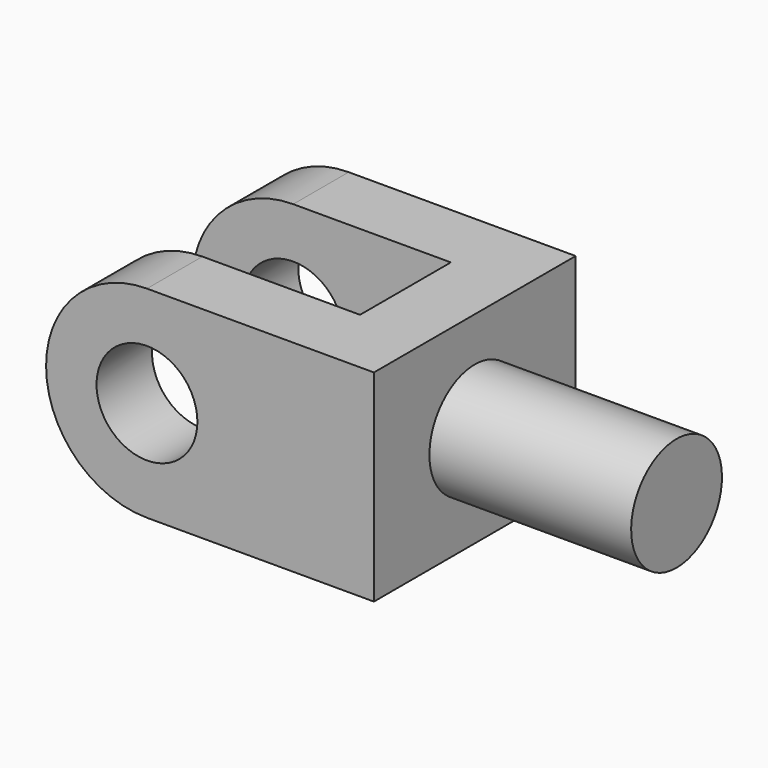
from build123d import *

# Parameters (mm, degrees)
F1_DEPTH = 812.8
F2_R     = 406.39999
F3_R     = 203.2
F4_DEPTH = 1016.001
F6_DEPTH = 812.8


# Not quite as in the source:
# - a fillet or chamfer is up to 0.001 mm smaller than in the source, because OpenCascade refuses the exact size


with BuildPart() as f1:
    # F0 (on Top) → F1 (new body)
    with BuildSketch(Plane.XY):
        Polygon((-69.4132745266, 217.2510341048), (-69.4132745266, -62.1489658952), (1251.3867254734, -62.1489658952), (1251.3867254734, 953.8510341048), (-69.4132745266, 953.8510341048), (-69.4132745266, 674.4510341048), (971.9867254734, 674.4510341048), (971.9867254734, 217.2510341048), align=None)
    extrude(amount=F1_DEPTH)

    # F2 (radius 406.4 in the source; OpenCascade refuses exactly that, so slightly less here)
    f2_edges = [f1.edges().sort_by_distance(p)[0] for p in [
        (-69.413275, 77.551034, 812.8),
        (-69.413275, 77.551034, 0),
        (-69.413275, 814.151034, 812.8),
        (-69.413275, 814.151034, 0),
    ]]
    fillet(f2_edges, radius=F2_R)

    # F3 (on face) → F4 (cut, through all)
    with BuildSketch(Plane.XZ.offset(62.1489658952)):
        with Locations((336.9867254734, 406.4)):
            Circle(F3_R)
    extrude(amount=-F4_DEPTH, mode=Mode.SUBTRACT)

    # F5 (on face) → F6 (join)
    with BuildSketch(Plane.YZ.offset(1251.3867254734)):
        with BuildLine():
            Line((445.8510341048, 177.8), (445.8510341048, 635))
            ThreePointArc((445.8510341048, 635), (217.2510341048, 406.4), (445.8510341048, 177.8))
        make_face()
        with BuildLine():
            ThreePointArc((674.4510341048, 406.4), (607.4956442841, 568.0446101792), (445.8510341048, 635))
            Line((445.8510341048, 635), (445.8510341048, 177.8))
            ThreePointArc((445.8510341048, 177.8), (607.4956442841, 244.7553898208), (674.4510341048, 406.4))
        make_face()
    extrude(amount=F6_DEPTH)


solid = f1.part
